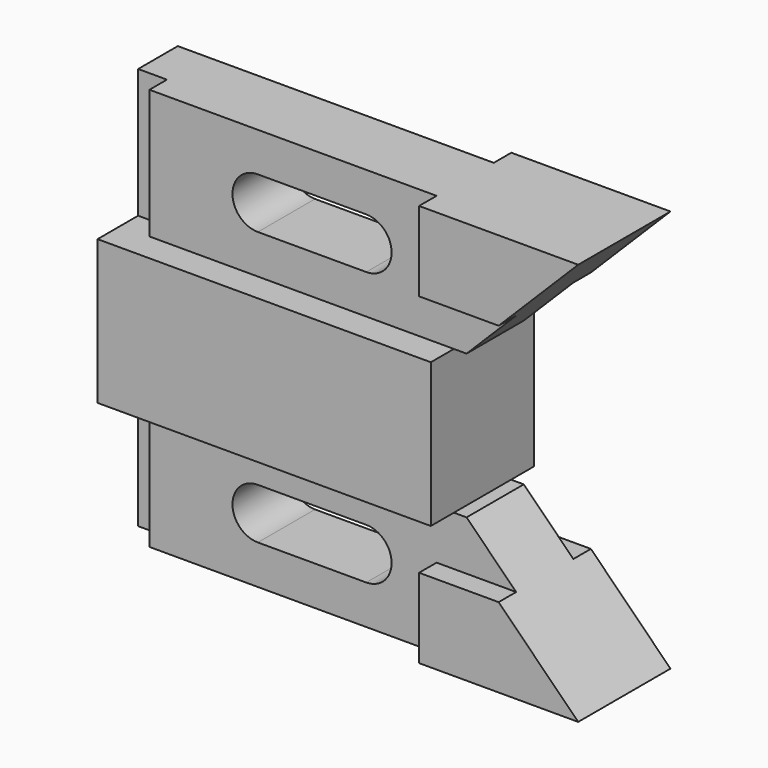
from build123d import *

# Parameters (mm, degrees)
F0_W          = 28.448
F0_H          = 31.75
F1_DEPTH      = 73.406
F3_DEPTH      = 7.874
F4_W          = 6.35
F4_H          = 28.448
F5_DEPTH      = 4.826
F6_DEPTH      = 4.826
F6_DEPTH_BACK = 20.574


# Not quite as in the source:
# - a pattern or mirror of a feature is missing from the dataset's text; its kind, count and spacing are read off the source's solid


with BuildPart() as f1:
    # F0 (on Right) → F1 (new body)
    with BuildSketch(Plane.YZ):
        Rectangle(F0_W, F0_H)
    extrude(amount=F1_DEPTH)

    # F2 (on Front) → F3 (join, symmetric)
    with BuildSketch(Plane.XZ):
        Polygon((0, 15.875), (73.406, 15.875), (76.2, 15.875), (104.648, 44.323), (0, 44.323), align=None)
        with BuildLine():
            ThreePointArc((30.226, 24.511), (24.638, 30.099), (30.226, 35.687))
            Line((30.226, 35.687), (54.102, 35.687))
            ThreePointArc((54.102, 35.687), (58.0533126933, 34.0503126933), (59.69, 30.099))
            ThreePointArc((59.69, 30.099), (58.0533126933, 26.1476873067), (54.102, 24.511))
            Line((54.102, 24.511), (30.226, 24.511))
        make_face(mode=Mode.SUBTRACT)
        Polygon((104.648, -44.323), (76.2, -15.875), (73.406, -15.875), (0, -15.875), (0, -44.323), align=None)
        with BuildLine():
            ThreePointArc((30.226, -35.687), (24.638, -30.099), (30.226, -24.511))
            Line((30.226, -24.511), (54.102, -24.511))
            ThreePointArc((54.102, -24.511), (58.0533126933, -26.1476873067), (59.69, -30.099))
            ThreePointArc((59.69, -30.099), (58.0533126933, -34.0503126933), (54.102, -35.687))
            Line((54.102, -35.687), (30.226, -35.687))
        make_face(mode=Mode.SUBTRACT)
    extrude(amount=F3_DEPTH, both=True)

    # F4 (on face) → F5 (cut)
    with BuildSketch(Plane.XZ.offset(7.874)):
        with Locations((3.175, 30.099)):
            Rectangle(F4_W, F4_H)
    f5 = extrude(amount=-F5_DEPTH, mode=Mode.SUBTRACT)

    # F5_copies: F5 across plane
    add(f5.mirror(Plane(origin=(0, 0, 0), x_dir=(-1, 0, 0), z_dir=(0, 0, -1))), mode=Mode.SUBTRACT)

    # F4 (on face) → F6 (join, two sides)
    with BuildSketch(Plane.XZ.offset(7.874)) as f6_sk:
        Polygon((104.648, 44.323), (69.596, 44.323), (69.596, 26.797), (87.122, 26.797), align=None)
    f6 = extrude(amount=F6_DEPTH) + extrude(f6_sk.sketch, amount=-F6_DEPTH_BACK)

    # F6_copies: F6 across plane
    add(f6.mirror(Plane(origin=(0, 0, 0), x_dir=(-1, 0, 0), z_dir=(0, 0, -1))))


solid = f1.part
